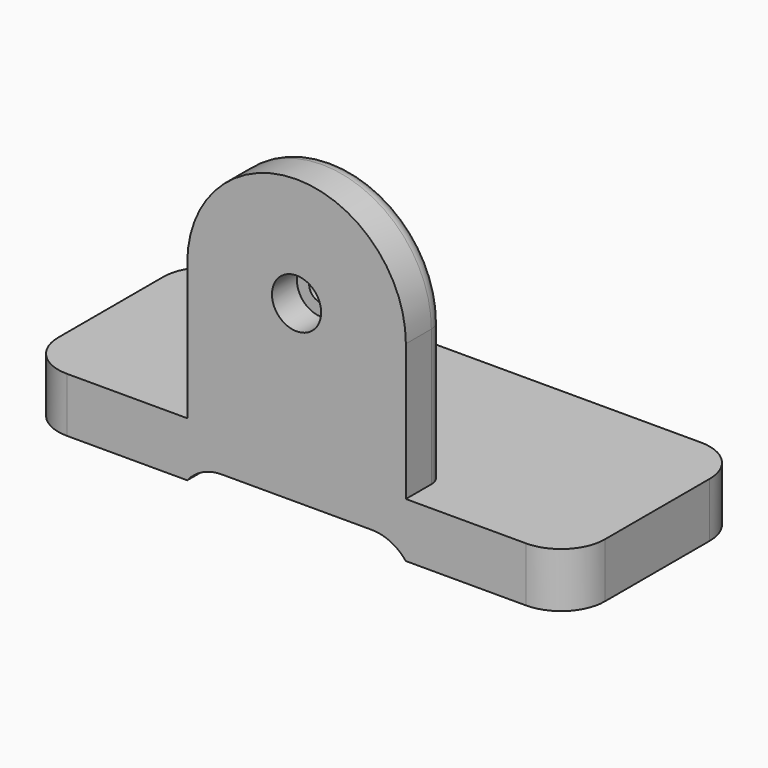
from build123d import *

# Parameters (mm, degrees)
F0_W         = 100
F0_H         = 40
F1_DEPTH     = 10
F3_DEPTH     = 8.82827
F4_W         = 40
F4_H         = 3
F5_DEPTH     = 40.001
F6_R         = 2.25
F7_DEPTH     = 40.001
F8_R         = 4.5
F9_DEPTH     = 5.7
F10_T1_DEPTH = 40
F10_T3_DEPTH = 50
F10_T5_DEPTH = 50
F10_T7_DEPTH = 50
F10_T9_DEPTH = 50
F11_T1_DEPTH = 40
F12_R        = 3


# Not quite as in the source:
# - a fillet or chamfer that OpenCascade refuses, or shapes differently, is made with other operations: its cross-section is extruded or revolved along the edge and cut away or added


with BuildPart() as f1:
    # F0 (on Top) → F1 (new body)
    with BuildSketch(Plane.XY):
        with Locations((-50, 20)):
            Rectangle(F0_W, F0_H)
    extrude(amount=F1_DEPTH)

    # F2 (on face) → F3 (join)
    with BuildSketch(Plane.XZ):
        with BuildLine():
            ThreePointArc((-30, 35), (-50, 55), (-70, 35))
            Line((-70, 35), (-70, 0))
            Line((-70, 0), (-30, 0))
            Line((-30, 0), (-30, 35))
        make_face()
    extrude(amount=-F3_DEPTH)

    # F4 (on Front) → F5 (cut, through all)
    with BuildSketch(Plane.XZ):
        with Locations((-50, 1.5)):
            Rectangle(F4_W, F4_H)
    extrude(amount=-F5_DEPTH, mode=Mode.SUBTRACT)

    # F6 (on face) → F7 (cut, through all)
    with BuildSketch(Plane.XZ):
        with Locations((-50, 35)):
            Circle(F6_R)
    extrude(amount=-F7_DEPTH, mode=Mode.SUBTRACT)

    # F8 (on face) → F9 (cut)
    with BuildSketch(Plane.XZ):
        with Locations((-50, 35)):
            Circle(F8_R)
    extrude(amount=-F9_DEPTH, mode=Mode.SUBTRACT)

    # F10: fillet of radius 8 on 5 edges, made by hand

    # F10_s2 → F10_t1 (join)
    with BuildSketch(Plane.XZ.offset(-40)):
        with BuildLine():
            ThreePointArc((-36.2449979984, 3), (-32.7808963833, 2.2111025509), (-30, 0))
            Line((-30, 0), (-30, 3))
            Line((-30, 3), (-36.2449979984, 3))
        make_face()
    extrude(amount=F10_T1_DEPTH)

    # F10_s4 → F10_t3 (cut)
    with BuildSketch(Plane.XY.offset(-20)):
        with BuildLine():
            ThreePointArc((-92, 0), (-97.6568542495, 2.3431457505), (-100, 8))
            Line((-100, 8), (-100, 0))
            Line((-100, 0), (-92, 0))
        make_face()
    extrude(amount=F10_T3_DEPTH, mode=Mode.SUBTRACT)

    # F10_s6 → F10_t5 (cut)
    with BuildSketch(Plane.XY.offset(-20)):
        with BuildLine():
            ThreePointArc((-8, 0), (-2.3431457505, 2.3431457505), (0, 8))
            Line((0, 8), (0, 0))
            Line((0, 0), (-8, 0))
        make_face()
    extrude(amount=F10_T5_DEPTH, mode=Mode.SUBTRACT)

    # F10_s8 → F10_t7 (cut)
    with BuildSketch(Plane.XY.offset(-20)):
        with BuildLine():
            ThreePointArc((-100, 32), (-97.6568542495, 37.6568542495), (-92, 40))
            Line((-92, 40), (-100, 40))
            Line((-100, 40), (-100, 32))
        make_face()
    extrude(amount=F10_T7_DEPTH, mode=Mode.SUBTRACT)

    # F10_s10 → F10_t9 (cut)
    with BuildSketch(Plane.XY.offset(-20)):
        with BuildLine():
            ThreePointArc((-8, 40), (-2.3431457505, 37.6568542495), (0, 32))
            Line((0, 32), (0, 40))
            Line((0, 40), (-8, 40))
        make_face()
    extrude(amount=F10_T9_DEPTH, mode=Mode.SUBTRACT)

    # F11: fillet of radius 8 on 1 edges, made by hand

    # F11_s2 → F11_t1 (join)
    with BuildSketch(Plane.XZ.offset(-40)):
        with BuildLine():
            ThreePointArc((-70, 0), (-67.2191036167, 2.2111025509), (-63.7550020016, 3))
            Line((-63.7550020016, 3), (-70, 3))
            Line((-70, 3), (-70, 0))
        make_face()
    extrude(amount=F11_T1_DEPTH)

    # F12
    f12_edges = [f1.edges().sort_by_distance(p)[0] for p in [
        (-50, 8.82827, 55),
        (-30, 8.82827, 22.5),
        (-70, 8.82827, 22.5),
    ]]
    fillet(f12_edges, radius=F12_R)


solid = f1.part
